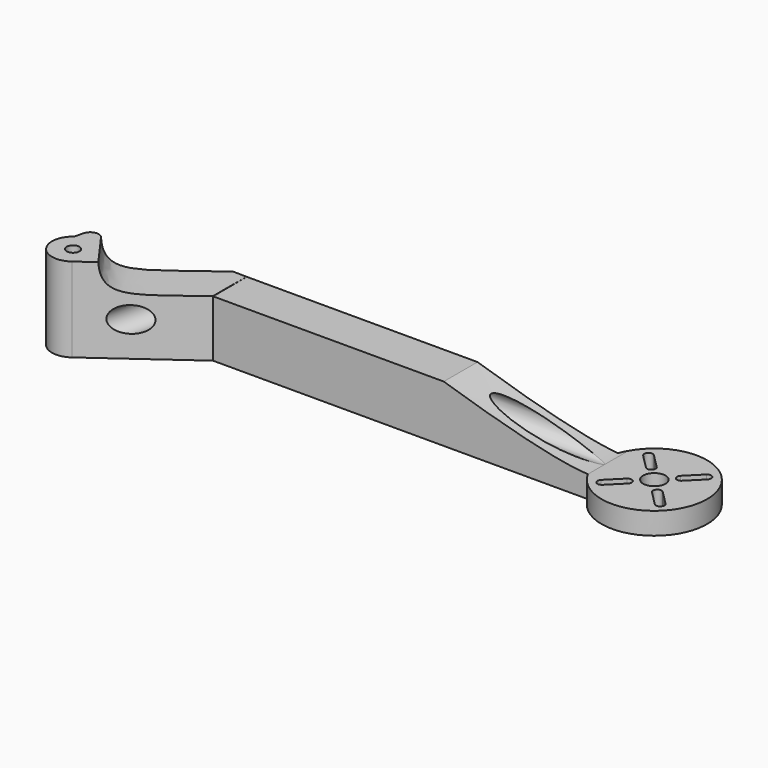
from build123d import *

# Parameters (mm, degrees)
F0_R          = 1.5
F0_R_2        = 2.6412895019
F1_DEPTH      = 20
F3_DEPTH      = 25
F3_DEPTH_BACK = 25
F5_DEPTH      = 25
F8_R          = 3
F11_DEPTH     = 20
F12_T1_DEPTH  = 41.4280655281


# Not quite as in the source:
# - a fillet or chamfer that OpenCascade refuses, or shapes differently, is made with other operations: its cross-section is extruded or revolved along the edge and cut away or added


with BuildPart() as f1:
    # F0 (on Top) → F1 (new body)
    with BuildSketch(Plane.XY):
        with BuildLine():
            Line((-136.9092201152, 53.1693232265), (-48.1315898414, 53.1693232265))
            ThreePointArc((-48.1315898414, 53.1693232265), (-24.7040865671, 60.2304450376), (-48.9954501741, 63.1693232265))
            Line((-48.9954501741, 63.1693232265), (-140.1388241649, 63.1693232265))
            Line((-140.1388241649, 63.1693232265), (-164.0276092996, 45.9422132412))
            ThreePointArc((-164.0276092996, 45.9422132412), (-165.0669659453, 38.947333564), (-158.0720862682, 37.9079769183))
            Line((-158.0720862682, 37.9079769183), (-136.9092201152, 53.1693232265))
        make_face()
        with Locations((-161.0498477839, 41.9250950797)):
            Circle(F0_R, mode=Mode.SUBTRACT)
        with BuildLine():
            ThreePointArc((-43.3736355328, 51.5244823211), (-44.7878490952, 51.5244823211), (-44.7878490952, 52.9386958835))
            Line((-44.7878490952, 52.9386958835), (-41.4003457692, 56.3261992095))
            ThreePointArc((-41.4003457692, 56.3261992095), (-39.9861322069, 56.3261992095), (-39.9861322069, 54.9119856471))
            Line((-39.9861322069, 54.9119856471), (-43.3736355328, 51.5244823211))
        make_face(mode=Mode.SUBTRACT)
        with BuildLine():
            ThreePointArc((-29.527561069, 52.9386958835), (-29.527561069, 51.5244823211), (-30.9417746314, 51.5244823211))
            Line((-30.9417746314, 51.5244823211), (-34.3292779574, 54.9119856471))
            ThreePointArc((-34.3292779574, 54.9119856471), (-34.3292779574, 56.3261992095), (-32.915064395, 56.3261992095))
            Line((-32.915064395, 56.3261992095), (-29.527561069, 52.9386958835))
        make_face(mode=Mode.SUBTRACT)
        with Locations((-37.1577050821, 59.1546263342)):
            Circle(F0_R_2, mode=Mode.SUBTRACT)
        with BuildLine():
            Line((-41.4003457692, 61.9830534589), (-44.7878490952, 65.3705567849))
            ThreePointArc((-44.7878490952, 65.3705567849), (-44.7878490952, 66.7847703473), (-43.3736355328, 66.7847703473))
            Line((-43.3736355328, 66.7847703473), (-39.9861322069, 63.3972670213))
            ThreePointArc((-39.9861322069, 63.3972670213), (-39.9861322069, 61.9830534589), (-41.4003457692, 61.9830534589))
        make_face(mode=Mode.SUBTRACT)
        with BuildLine():
            ThreePointArc((-30.9417746314, 66.7847703473), (-29.527561069, 66.7847703473), (-29.527561069, 65.3705567849))
            Line((-29.527561069, 65.3705567849), (-32.915064395, 61.9830534589))
            ThreePointArc((-32.915064395, 61.9830534589), (-34.3292779574, 61.9830534589), (-34.3292779574, 63.3972670213))
            Line((-34.3292779574, 63.3972670213), (-30.9417746314, 66.7847703473))
        make_face(mode=Mode.SUBTRACT)
    extrude(amount=F1_DEPTH)

    # F2 (on face) → F3 (cut, two sides)
    with BuildSketch(Plane.XZ.offset(-53.1693232265)) as f3_sk:
        with BuildLine():
            add(Edge.make_bspline(
                [(-48.1315898414, 5.1997262053), (-55.5737955735, 5.517366778), (-70.0693075174, 9.5402547737), (-82.2478533544, 13.4277092293)],
                knots=[0, 0, 0, 0, 32.5655157772, 32.5655157772, 32.5655157772, 32.5655157772], degree=3))
            Line((-48.1315898414, 5.1997262053), (-22.6805435396, 5.1997262053))
            Line((-22.6805435396, 5.1997262053), (-24.4416198375, 23.0218202323))
            Line((-24.4416198375, 23.0218202323), (-102.9450073838, 23.9689107984))
            Line((-102.9450073838, 23.9689107984), (-109.8586171865, 20))
            Line((-109.8586171865, 20), (-136.9092201152, 24.3437178433))
            Line((-136.9092201152, 24.3437178433), (-136.9092201152, 13.4277092293))
            Line((-136.9092201152, 13.4277092293), (-82.2478533544, 13.4277092293))
        make_face()
    extrude(amount=-F3_DEPTH, mode=Mode.SUBTRACT)
    extrude(f3_sk.sketch, amount=F3_DEPTH_BACK, mode=Mode.SUBTRACT)

    # F4 (on face) → F5 (cut)
    with BuildSketch(Plane(origin=(-77.913469167, 108.0423893277, 0), x_dir=(-0.8110964415, -0.5849124402, 0), z_dir=(-0.5849124402, 0.8110964415, 0))):
        with BuildLine():
            Line((73.6283713512, 25.1456971396), (74.0980582459, 13.4277092293))
            add(Edge.make_bspline(
                [(74.0980582459, 13.4277092293), (92.9379910232, 13.834843412), (100.7777675986, 11.1937364563), (101.1828109622, 20)],
                knots=[0, 0, 0, 0, 27.8707523342, 27.8707523342, 27.8707523342, 27.8707523342], degree=3))
            Line((101.1828109622, 20), (97.8787563539, 26.1177145299))
            Line((97.8787563539, 26.1177145299), (73.6283713512, 25.1456971396))
        make_face()
    extrude(amount=-F5_DEPTH, mode=Mode.SUBTRACT)

    # F9: sweep along a path in F6
    with BuildLine(Plane.XY.offset(5.1997262053)) as f9_path:
        Line((-61.2067505717, 58.1693232265), (-86.7135846391, 58.1693232265))
        Line((-86.7135846391, 58.1693232265), (-137.850685735, 58.1693232265))
        Line((-137.850685735, 58.1693232265), (-147.6771980524, 50.9236194193))
        Line((-147.6771980524, 50.9236194193), (-156.9756269455, 10.3533519432))
    # F8 (on face) → F9 (sweep, cut)
    with BuildSketch(Plane.YZ.offset(-48.1315898414)):
        with Locations((58.2011528313, 8.1997262053)):
            Circle(F8_R)
    sweep(path=f9_path.line, transition=Transition.RIGHT, mode=Mode.SUBTRACT)

    # F10 (on face) → F11 (join)
    with BuildSketch(Plane(origin=(0, 0, 0), x_dir=(1, 0, 0), z_dir=(0, 0, -1))):
        Polygon((-159.9824870749, -48.8593044651), (-164.0276092996, -45.9422132412), (-162.4302172451, -52.2535650319), align=None)
    extrude(amount=-F11_DEPTH)

    # F12: fillet of radius 2 on 1 edges, made by hand

    # F12_s2 → F12_t1 (cut)
    with BuildSketch(Plane.XY.offset(-10.7140327641)):
        with BuildLine():
            ThreePointArc((-163.4817415016, 48.0989559734), (-161.9675459982, 49.5626274076), (-159.9824870749, 48.8593044651))
            Line((-159.9824870749, 48.8593044651), (-162.4302172451, 52.2535650319))
            Line((-162.4302172451, 52.2535650319), (-163.4817415016, 48.0989559734))
        make_face()
    extrude(amount=F12_T1_DEPTH, mode=Mode.SUBTRACT)


solid = f1.part
